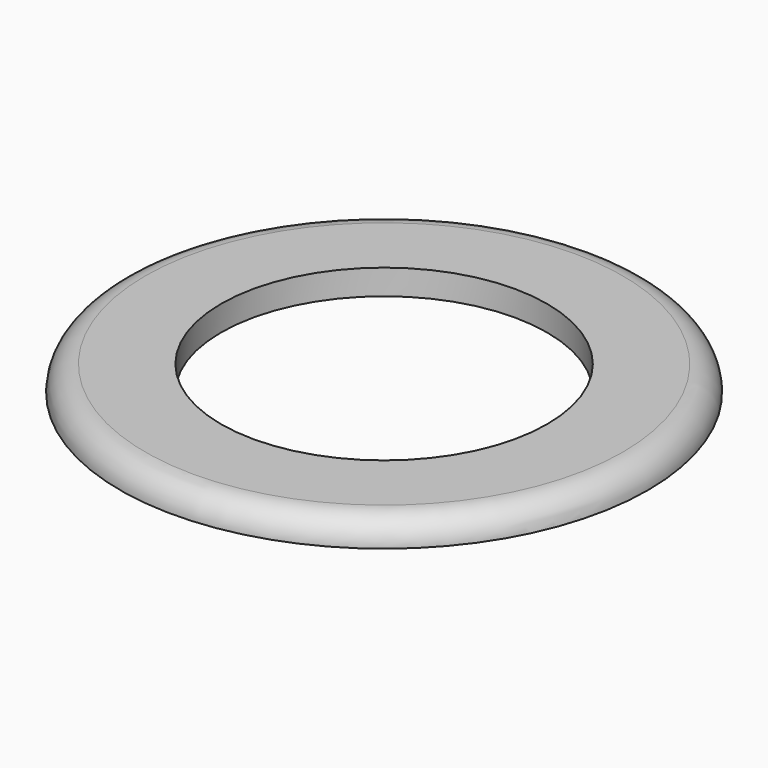
from build123d import *

# Parameters (mm, degrees)
F0_R     = 66.421
F0_R_2   = 41.021
F1_DEPTH = 6.35
F2_R     = 6.34999


# Not quite as in the source:
# - a fillet or chamfer is up to 0.001 mm smaller than in the source, because OpenCascade refuses the exact size


with BuildPart() as f1:
    # F0 (on Top) → F1 (new body)
    with BuildSketch(Plane.XY):
        Circle(F0_R)
        Circle(F0_R_2, mode=Mode.SUBTRACT)
    extrude(amount=F1_DEPTH)

    # F2 (radius 6.35 in the source; OpenCascade refuses exactly that, so slightly less here)
    f2_edges = [f1.edges().sort_by_distance(p)[0] for p in [
        (-66.421, 0, 6.35),
    ]]
    fillet(f2_edges, radius=F2_R)


solid = f1.part
